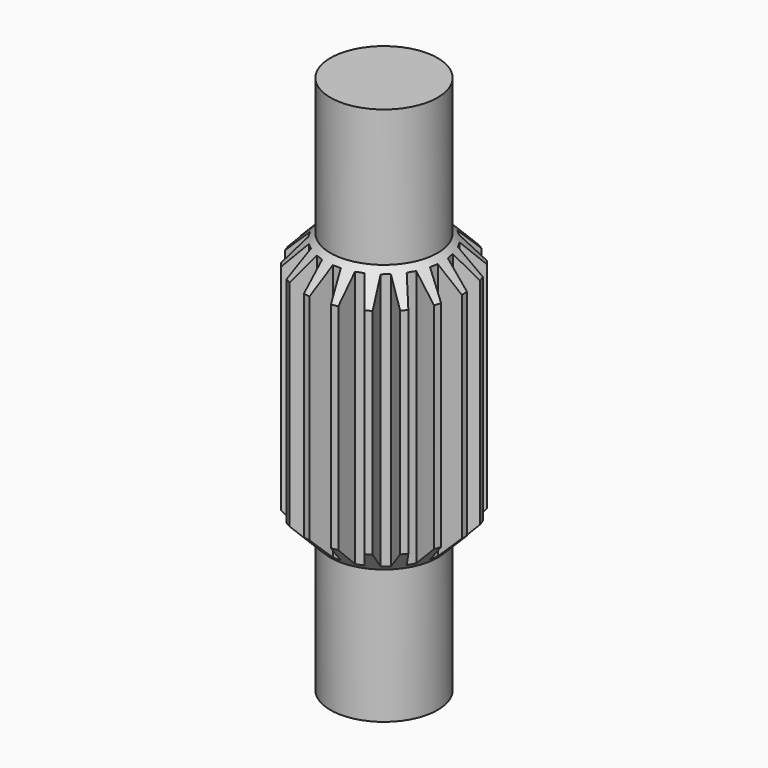
from build123d import *

# Parameters (mm, degrees)
F0_R            = 7.62
F1_DEPTH        = 25.4
F2_SIZE         = 2.54
F4_DEPTH        = 25.4
F4_COPIES_COUNT = 18
F6_R            = 5.08
F7_DEPTH        = 12.954
F8_R            = 5.08
F9_DEPTH        = 12.7


# Not quite as in the source:
# - a pattern or mirror of a feature is missing from the dataset's text; its kind, count and spacing are read off the source's solid


with BuildPart() as f1:
    # F0 (on Top) → F1 (new body)
    with BuildSketch(Plane.XY):
        Circle(F0_R)
    extrude(amount=F1_DEPTH)

    # F2
    f2_edges = [f1.edges().sort_by_distance(p)[0] for p in [
        (-7.62, 0, 25.4),
        (-7.62, 0, 0),
    ]]
    chamfer(f2_edges, length=F2_SIZE)

    # F3 (on face) → F4 (cut, through all)
    with BuildSketch(Plane.XY.offset(25.4)):
        with BuildLine():
            ThreePointArc((1.016, 7.5519629236), (0, 7.62), (-1.016, 7.5519629236))
            Line((-1.016, 7.5519629236), (-0.381, 5.588))
            Line((-0.381, 5.588), (0.381, 5.588))
            Line((0.381, 5.588), (1.016, 7.5519629236))
        make_face()
    f4 = extrude(amount=-F4_DEPTH, mode=Mode.SUBTRACT)

    # F4_copies: F4 ×18 about axis
    f4_copies_axis = Axis((0, 0, 0), (0, 0, 1))
    for i in range(1, F4_COPIES_COUNT):
        add(f4.rotate(f4_copies_axis, i * 360 / F4_COPIES_COUNT), mode=Mode.SUBTRACT)

    # F6 (on face) → F7 (join)
    with BuildSketch(Plane.XY.offset(25.4)):
        Circle(F6_R)
    extrude(amount=F7_DEPTH)

    # F8 (on face) → F9 (join)
    with BuildSketch(Plane(origin=(0, 0, 0), x_dir=(1, 0, 0), z_dir=(0, 0, -1))):
        Circle(F8_R)
    extrude(amount=F9_DEPTH)


solid = f1.part
